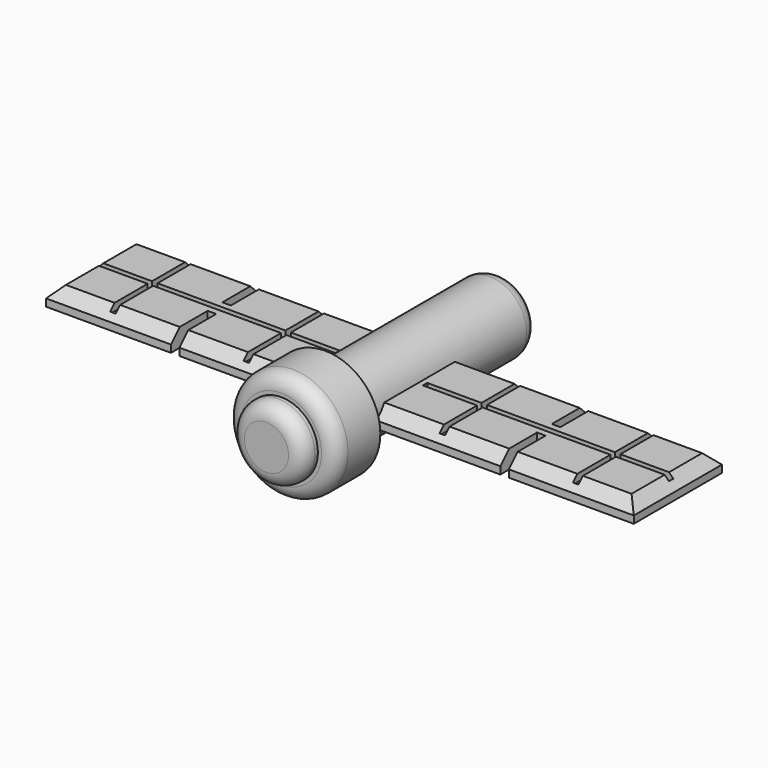
from build123d import *

# Parameters (mm, degrees)
F1_R          = 12.7
F2_DEPTH      = 101.6
F3_R          = 5.08
F4_W          = 38.1
F4_H          = 6.35
F5_DEPTH      = 101.6
F6_DEPTH      = 101.6
F7_W          = 2.9432778758
F7_H          = 15.875
F8_DEPTH      = 25.4
F9_W          = 2.9432778758
F9_H          = 15.875
F10_DEPTH     = 25.4
F11_W         = 1.905
F11_H         = 16.1925
F11_W_2       = 18.7325
F11_H_2       = 1.905
F11_W_3       = 44.2182778758
F11_W_4       = 1.8969494015
F11_W_5       = 18.7405505985
F12_DEPTH     = 2.54
F13_W         = 18.7325
F13_H         = 1.905
F13_W_2       = 1.9137861806
F13_H_2       = 16.1925
F13_W_3       = 44.2094916952
F13_W_4       = 1.905
F13_W_5       = 18.3292221242
F14_DEPTH     = 2.54
F15_T1_DEPTH  = 57.6962243683
F15_T3_DEPTH  = 62.7762243683
F15_T5_DEPTH  = 62.7762243683
F15_T10_DEPTH = 62.7762243683
F15_S11_R     = 12.7
F15_T12_DEPTH = 33
F15_T16_DEPTH = 62.7762243683
F15_S17_R     = 12.7
F15_T18_DEPTH = 33
F15_T22_DEPTH = 62.7762243683
F15_S23_R     = 12.7
F15_T24_DEPTH = 33
F15_T28_DEPTH = 62.7762243683
F15_S29_R     = 12.7
F15_T30_DEPTH = 33
F17_R         = 19.05
F18_DEPTH     = 19.05
F19_R         = 5.08


# Not quite as in the source:
# - a fillet or chamfer that OpenCascade refuses, or shapes differently, is made with other operations: its cross-section is extruded or revolved along the edge and cut away or added


with BuildPart() as f2:
    # F1 (on offset) → F2 (new body)
    with BuildSketch(Plane.XZ.offset(50.8)):
        Circle(F1_R)
    extrude(amount=-F2_DEPTH)

    # F3
    f3_edges = [f2.edges().sort_by_distance(p)[0] for p in [
        (-12.7, -50.8, 0),
        (-12.7, 50.8, 0),
    ]]
    fillet(f3_edges, radius=F3_R)

    # F4 (on Right) → F5 (join)
    with BuildSketch(Plane.YZ):
        Rectangle(F4_W, F4_H)
    extrude(amount=F5_DEPTH)

    # F4 (on Right) → F6 (join)
    with BuildSketch(Plane.YZ):
        Rectangle(F4_W, F4_H)
    extrude(amount=-F6_DEPTH)

    # F7 (on face) → F8 (cut)
    with BuildSketch(Plane.XY.offset(3.175)):
        with Locations((-56.9483610621, 11.1125)):
            Rectangle(F7_W, F7_H)
        with Locations((-56.9483610621, -11.1125)):
            Rectangle(F7_W, F7_H)
    extrude(amount=-F8_DEPTH, mode=Mode.SUBTRACT)

    # F9 (on face) → F10 (cut)
    with BuildSketch(Plane.XY.offset(3.175)):
        with Locations((56.9483610621, 11.1125)):
            Rectangle(F9_W, F9_H)
        with Locations((56.9483610621, -11.1125)):
            Rectangle(F9_W, F9_H)
    extrude(amount=-F10_DEPTH, mode=Mode.SUBTRACT)

    # F11 (on face) → F12 (cut)
    with BuildSketch(Plane.XY.offset(3.175)):
        with Locations((-80.01, 9.04875)):
            Rectangle(F11_W, F11_H)
        with Locations((-90.32875, 0)):
            Rectangle(F11_W_2, F11_H_2)
        with Locations((-80.01, 0)):
            Rectangle(F11_W, F11_H_2)
        with Locations((-80.01, -9.04875)):
            Rectangle(F11_W, F11_H)
        with Locations((-56.9483610621, 0)):
            Rectangle(F11_W_3, F11_H_2)
        with Locations((-33.8907474235, -9.04875)):
            Rectangle(F11_W_4, F11_H)
        with Locations((-33.8907474235, 0)):
            Rectangle(F11_W_4, F11_H_2)
        with Locations((-33.8907474235, 9.04875)):
            Rectangle(F11_W_4, F11_H)
        with Locations((-23.5719974235, 0)):
            Rectangle(F11_W_5, F11_H_2)
    extrude(amount=-F12_DEPTH, mode=Mode.SUBTRACT)

    # F13 (on face) → F14 (cut)
    with BuildSketch(Plane.XY.offset(3.175)):
        with Locations((23.5679721242, 0)):
            Rectangle(F13_W, F13_H)
        with Locations((33.8911152145, 9.04875)):
            Rectangle(F13_W_2, F13_H_2)
        with Locations((33.8911152145, 0)):
            Rectangle(F13_W_2, F13_H)
        with Locations((33.8911152145, -9.04875)):
            Rectangle(F13_W_2, F13_H_2)
        with Locations((56.9527541524, 0)):
            Rectangle(F13_W_3, F13_H)
        with Locations((80.01, 9.04875)):
            Rectangle(F13_W_4, F13_H_2)
        with Locations((80.01, 0)):
            Rectangle(F13_W_4, F13_H)
        with Locations((90.1271110621, 0)):
            Rectangle(F13_W_5, F13_H)
        with Locations((80.01, -9.04875)):
            Rectangle(F13_W_4, F13_H_2)
    extrude(amount=-F14_DEPTH, mode=Mode.SUBTRACT)

    # F15: chamfer of 3.81 on 10 edges, made by hand

    # F15_s2 → F15_t1 (cut)
    with BuildSketch(Plane.XZ.offset(-28.8481121842)):
        Polygon((-97.79, 3.175), (-101.6, -0.635), (-101.6, 3.175), align=None)
        Polygon((97.79, 3.175), (101.6, -0.635), (101.6, 3.175), align=None)
    extrude(amount=F15_T1_DEPTH, mode=Mode.SUBTRACT)

    # F15_s4 → F15_t3 (cut)
    with BuildSketch(Plane.YZ.offset(48.6218878158)):
        Polygon((15.24, 3.175), (19.05, -0.635), (19.05, 3.175), align=None)
        Polygon((-15.24, 3.175), (-19.05, -0.635), (-19.05, 3.175), align=None)
    extrude(amount=F15_T3_DEPTH, mode=Mode.SUBTRACT)

    # F15_s6 → F15_t5 (cut)
    with BuildSketch(Plane.YZ.offset(-111.3981121842)):
        Polygon((-15.24, 3.175), (-19.05, -0.635), (-19.05, 3.175), align=None)
        Polygon((15.24, 3.175), (19.05, -0.635), (19.05, 3.175), align=None)
    extrude(amount=F15_T5_DEPTH, mode=Mode.SUBTRACT)


with BuildPart() as f15_tool8:
    # F15_s9 → F15_t10 (new body)
    with BuildSketch(Plane.YZ.offset(2.4986099401)):
        Polygon((19.05, -0.635), (15.24, 3.175), (19.05, 3.175), align=None)
    extrude(amount=F15_T10_DEPTH)

    # F15_s11 → F15_t12 (cut, symmetric)
    with BuildSketch(Plane.XZ.offset(-17.1)):
        Circle(F15_S11_R)
    extrude(amount=F15_T12_DEPTH, both=True, mode=Mode.SUBTRACT)


with BuildPart() as f2_1:
    add(f2.part)

    # F15_t7: cut F15_tool8
    add(f15_tool8.part, mode=Mode.SUBTRACT)


with BuildPart() as f15_tool14:
    # F15_s15 → F15_t16 (new body)
    with BuildSketch(Plane.YZ.offset(2.4986099401)):
        Polygon((-19.05, -0.635), (-15.24, 3.175), (-19.05, 3.175), align=None)
    extrude(amount=F15_T16_DEPTH)

    # F15_s17 → F15_t18 (cut, symmetric)
    with BuildSketch(Plane.XZ.offset(17.1)):
        Circle(F15_S17_R)
    extrude(amount=F15_T18_DEPTH, both=True, mode=Mode.SUBTRACT)


with BuildPart() as f2_2:
    add(f2_1.part)

    # F15_t13: cut F15_tool14
    add(f15_tool14.part, mode=Mode.SUBTRACT)


with BuildPart() as f15_tool20:
    # F15_s21 → F15_t22 (new body)
    with BuildSketch(Plane.YZ.offset(-2.4986099401)):
        Polygon((-19.05, -0.635), (-15.24, 3.175), (-19.05, 3.175), align=None)
    extrude(amount=-F15_T22_DEPTH)

    # F15_s23 → F15_t24 (cut, symmetric)
    with BuildSketch(Plane.XZ.offset(17.1)):
        Circle(F15_S23_R)
    extrude(amount=F15_T24_DEPTH, both=True, mode=Mode.SUBTRACT)


with BuildPart() as f2_3:
    add(f2_2.part)

    # F15_t19: cut F15_tool20
    add(f15_tool20.part, mode=Mode.SUBTRACT)


with BuildPart() as f15_tool26:
    # F15_s27 → F15_t28 (new body)
    with BuildSketch(Plane.YZ.offset(-2.4986099401)):
        Polygon((19.05, -0.635), (15.24, 3.175), (19.05, 3.175), align=None)
    extrude(amount=-F15_T28_DEPTH)

    # F15_s29 → F15_t30 (cut, symmetric)
    with BuildSketch(Plane.XZ.offset(-17.1)):
        Circle(F15_S29_R)
    extrude(amount=F15_T30_DEPTH, both=True, mode=Mode.SUBTRACT)


with BuildPart() as f2_4:
    add(f2_3.part)

    # F15_t25: cut F15_tool26
    add(f15_tool26.part, mode=Mode.SUBTRACT)

    # F17 (on offset) → F18 (join)
    with BuildSketch(Plane.XZ.offset(25.4)):
        Circle(F17_R)
    extrude(amount=F18_DEPTH)

    # F19
    f19_edges = [f2_4.edges().sort_by_distance(p)[0] for p in [
        (-19.05, -44.45, 0),
        (-7.62, -50.8, 0),
    ]]
    fillet(f19_edges, radius=F19_R)


solid = f2_4.part
